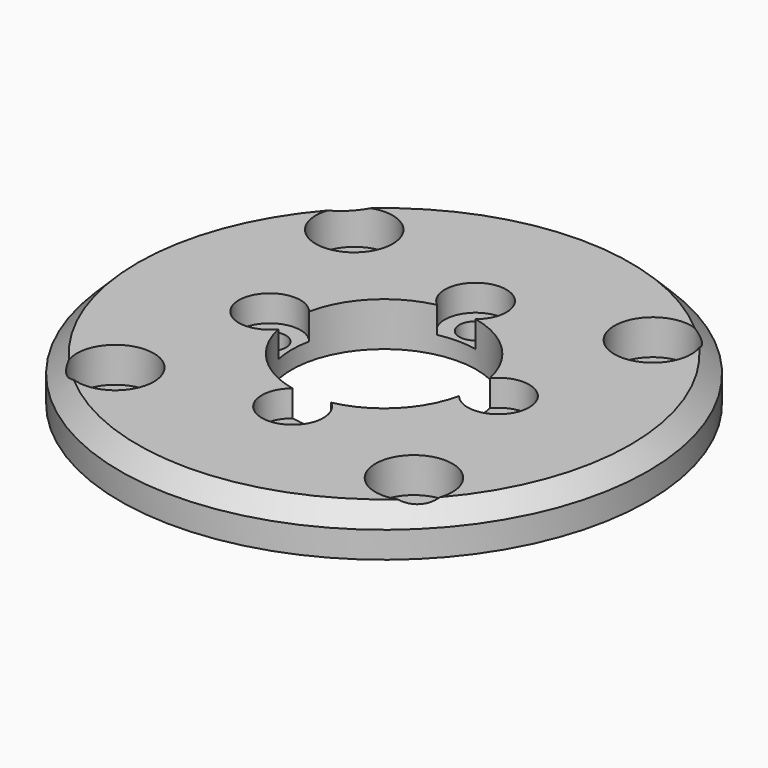
from build123d import *

# Parameters (mm, degrees)
F0_R           = 30
F0_R_2         = 10.5
F1_DEPTH       = 5
F3_D           = 4.7
F3_CBORE_D     = 8.75
F3_CBORE_DEPTH = 4
F5_D           = 3.7
F5_CBORE_D     = 7
F5_CBORE_DEPTH = 3


# Not quite as in the source:
# - a fillet or chamfer that OpenCascade refuses, or shapes differently, is made with other operations: its cross-section is extruded or revolved along the edge and cut away or added


with BuildPart() as f1:
    # F0 (on Top) → F1 (new body)
    with BuildSketch(Plane.XY):
        Circle(F0_R)
        Circle(F0_R_2, mode=Mode.SUBTRACT)
    extrude(amount=F1_DEPTH)

    # F3 (through all)
    with Locations(Plane.XY.offset(5)):
        with Locations((-16.9705627485, 16.9705627485), (16.9705627485, 16.9705627485), (16.9705627485, -16.9705627485), (-16.9705627485, -16.9705627485)):
            CounterBoreHole(F3_D / 2, F3_CBORE_D / 2, F3_CBORE_DEPTH)

    # F5 (through all)
    with Locations(Plane.XY.offset(5)):
        with Locations((0, 13), (-13, 0), (0, -13), (13, 0)):
            CounterBoreHole(F5_D / 2, F5_CBORE_D / 2, F5_CBORE_DEPTH)

    # F6: chamfer of 2 on 1 edges, made by hand

    # F6_s1 → F6_t2 (revolve, cut)
    with BuildSketch(Plane.XZ):
        Polygon((30, 3), (28, 5), (30, 5), align=None)
    revolve(axis=Axis((0, 0, 5), (0, 0, 1)), mode=Mode.SUBTRACT)


solid = f1.part
